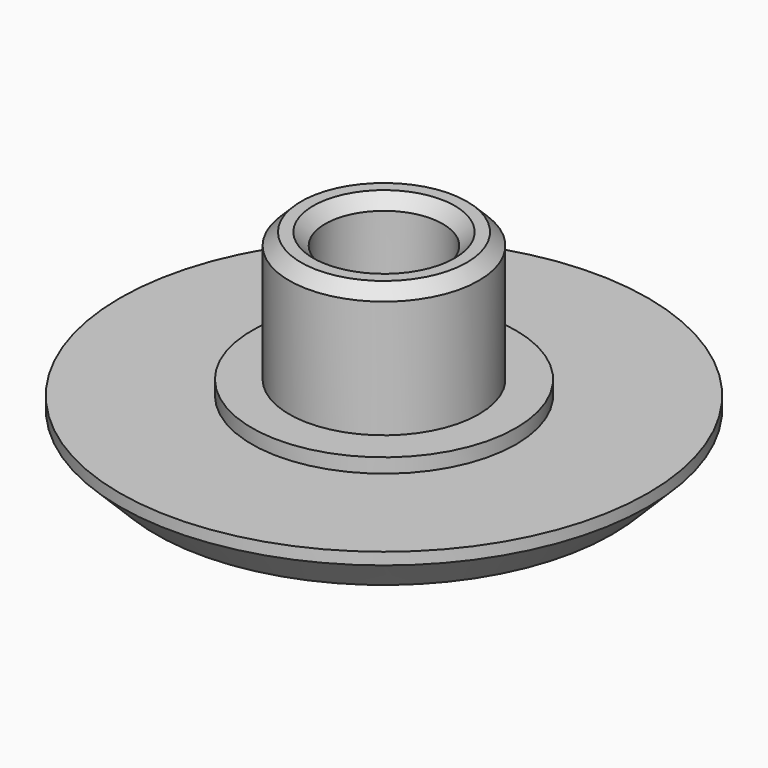
from build123d import *

# Parameters (mm, degrees)
F0_R     = 11
F0_R_2   = 5.5
F0_R_3   = 3.95
F0_R_4   = 2.45
F1_DEPTH = 2
F2_DEPTH = 2.6
F3_DEPTH = 8
F4_SIZE  = 0.5
F5_SIZE  = 0.5
F6_SIZE  = 1.5
F7_SIZE  = 1


# Not quite as in the source:
# - a feature names something its author has since deleted; it is built from what else it names


with BuildPart() as f1:
    # F0 (on Top) → F1 (new body)
    with BuildSketch(Plane.XY):
        Circle(F0_R)
        Circle(F0_R_2, mode=Mode.SUBTRACT)
        Circle(F0_R_2)
        Circle(F0_R_3, mode=Mode.SUBTRACT)
        Circle(F0_R_3)
        Circle(F0_R_4, mode=Mode.SUBTRACT)
        Circle(F0_R_4)
    extrude(amount=F1_DEPTH)

    # F0 (on Top) → F2 (join)
    with BuildSketch(Plane.XY):
        Circle(F0_R_2)
        Circle(F0_R_3, mode=Mode.SUBTRACT)
        Circle(F0_R_3)
        Circle(F0_R_4, mode=Mode.SUBTRACT)
        Circle(F0_R_4)
    extrude(amount=F2_DEPTH)

    # F0 (on Top) → F3 (join)
    with BuildSketch(Plane.XY):
        Circle(F0_R_3)
        Circle(F0_R_4, mode=Mode.SUBTRACT)
    extrude(amount=F3_DEPTH)

    # F4
    f4_edges = [f1.edges().sort_by_distance(p)[0] for p in [
        (-2.45, 0, 8),
    ]]
    chamfer(f4_edges, length=F4_SIZE)

    # F5
    f5_edges = [f1.edges().sort_by_distance(p)[0] for p in [
        (-3.95, 0, 8),
    ]]
    chamfer(f5_edges, length=F5_SIZE)

    # F6
    f6_edges = [f1.edges().sort_by_distance(p)[0] for p in [
        (-11, 0, 0),
    ]]
    chamfer(f6_edges, length=F6_SIZE)

    # F7
    f7_edges = [f1.edges().sort_by_distance(p)[0] for p in [
        (-2.45, 0, 2.6),
    ]]
    chamfer(f7_edges, length=F7_SIZE)


solid = f1.part
